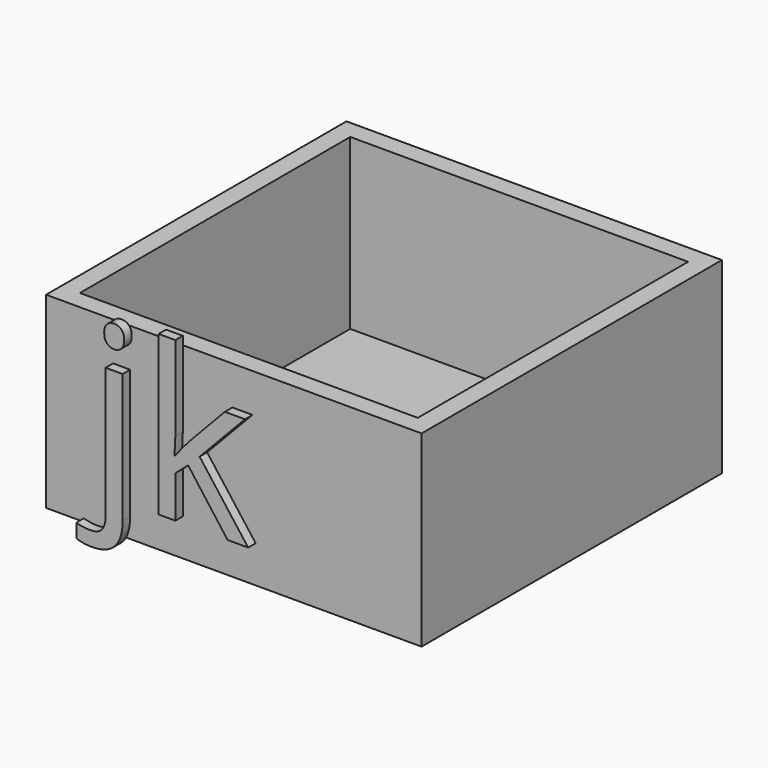
from build123d import *

# Parameters (mm, degrees)
F0_W         = 50.8
F0_H         = 25.4
F1_DEPTH     = 50.8
F2_T         = -2.54
F3_TEXT_SIZE = 28.3052101338
F4_DEPTH     = 1.27


# Not quite as in the source:
# - Text() gives the source's letters only with a copy of the font that has no kerning and outlines rounded to 1/6400 em; it was checked with that copy


with BuildPart() as f1:
    # F0 (on Front) → F1 (new body)
    with BuildSketch(Plane.XZ):
        with Locations((-15.5447140992, 16.0561242744)):
            Rectangle(F0_W, F0_H)
    extrude(amount=F1_DEPTH)

    # F2
    f2_openings = [f1.faces().sort_by_distance(p)[0] for p in [
        (-15.544714, -25.4, 28.756124),
    ]]
    offset(amount=F2_T, openings=f2_openings)

    # F3 (on face) → F4 (join)
    with BuildSketch(Plane.XZ.offset(50.8)):
        with Locations((-34.3025773764, 8.3763729781)):
            Text('jk', F3_TEXT_SIZE, font='Open Sans', text_align=(TextAlign.LEFT, TextAlign.BOTTOM))
    extrude(amount=F4_DEPTH)


solid = f1.part
